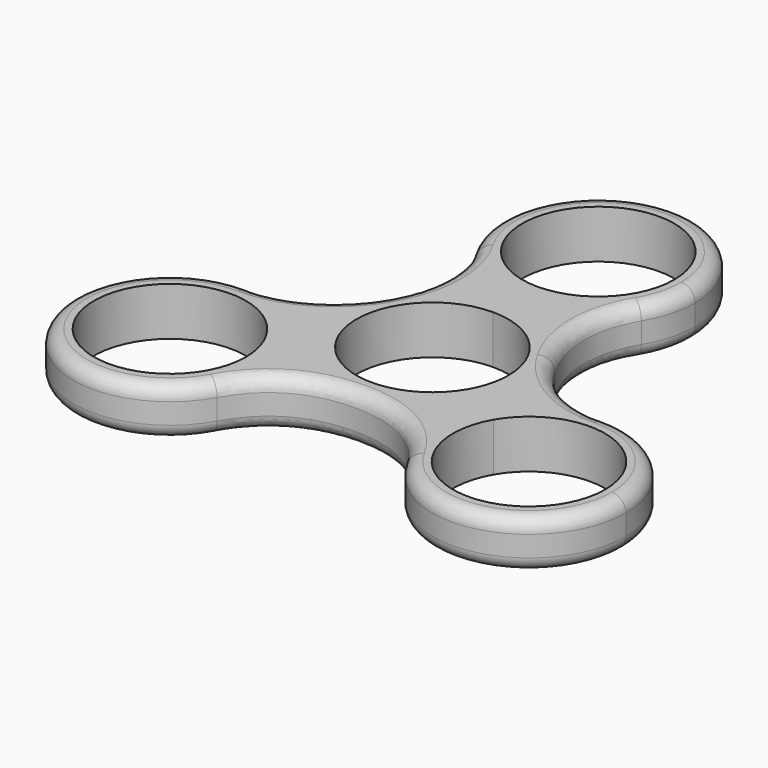
from build123d import *

# Parameters (mm, degrees)
F1_DEPTH = 7
F2_R     = 2


with BuildPart() as f1:
    # F0 (on Top) → F1 (new body)
    with BuildSketch(Plane.XY):
        with BuildLine():
            ThreePointArc((-11.9807621135, -15), (-12.4578005455, -11.3765333686), (-13.8564064606, -8))
            ThreePointArc((-13.8564064606, -8), (-18.8749387967, -2.9373603639), (-25.7357641151, -1.0021438791))
            ThreePointArc((-25.7357641151, -1.0021438791), (-38.1051177665, -22), (-13.7357641151, -21.7867535699))
            ThreePointArc((-13.7357641151, -21.7867535699), (-12.4266119746, -18.5049984324), (-11.9807621135, -15))
        make_face()
        with BuildLine():
            ThreePointArc((-14.9807621135, -15), (-36.6059462027, -17.8470094961), (-16.4544826719, -9.5))
            ThreePointArc((-16.4544826719, -9.5), (-15.3555780244, -12.1529905039), (-14.9807621135, -15))
        make_face(mode=Mode.SUBTRACT)
        with BuildLine():
            ThreePointArc((-9.5262794416, -5.5), (-9.5262794416, 5.5), (0, 11))
            Line((0, 11), (0, 14))
            ThreePointArc((0, 14), (-7.0000000057, 12.1243556497), (-12.1243556595, 6.9999999886))
            ThreePointArc((-12.1243556595, 6.9999999886), (-14, -6.6e-09), (-12.124355653, -7))
            Line((-12.124355653, -7), (-9.5262794416, -5.5))
        make_face()
        with BuildLine():
            Line((-13.8564064606, -8), (-12.124355653, -7))
            ThreePointArc((-12.124355653, -7), (-14, -6.6e-09), (-12.1243556595, 6.9999999886))
            add(Edge.make_bspline(
                [(-12.124355653, 7), (-14.8604643909, 2.2609206509), (-19.9785749652, -1.1029092968), (-25.7357641151, -1.0021438791)],
                knots=[0.5, 0.5, 0.5, 0.5, 1, 1, 1, 1], degree=3))
            ThreePointArc((-25.7357641151, -1.0021438791), (-18.8749387967, -2.9373603639), (-13.8564064606, -8))
        make_face()
        with BuildLine():
            Line((12.124355653, -7), (9.5262794416, -5.5))
            ThreePointArc((9.5262794416, -5.5), (0, -11), (-9.5262794416, -5.5))
            Line((-9.5262794416, -5.5), (-12.124355653, -7))
            ThreePointArc((-12.124355653, -7), (-6.9999999959, -12.1243556553), (9.4e-09, -14))
            ThreePointArc((9.4e-09, -14), (7.0000000041, -12.1243556506), (12.124355653, -7))
        make_face()
        with BuildLine():
            ThreePointArc((9.4e-09, -14), (-6.9999999959, -12.1243556553), (-12.124355653, -7))
            Line((-12.124355653, -7), (-13.8564064606, -8))
            ThreePointArc((-13.8564064606, -8), (-12.4578005455, -11.3765333686), (-11.9807621135, -15))
            ThreePointArc((-11.9807621135, -15), (-12.4266119746, -18.5049984324), (-13.7357641151, -21.7867535699))
            add(Edge.make_bspline(
                [(-13.7357641151, -21.7867535699), (-10.4992239257, -15.947226949), (-5.2496119628, -14), (0, -14)],
                knots=[0, 0, 0, 0, 0.5, 0.5, 0.5, 0.5], degree=3))
        make_face()
        with BuildLine():
            Line((13.8564064606, -8), (12.124355653, -7))
            ThreePointArc((12.124355653, -7), (7.0000000041, -12.1243556506), (9.4e-09, -14))
            add(Edge.make_bspline(
                [(0, -14), (5.2496119628, -14), (10.4992239257, -15.947226949), (13.7357641151, -21.7867535699)],
                knots=[0.5, 0.5, 0.5, 0.5, 1, 1, 1, 1], degree=3))
            ThreePointArc((13.7357641151, -21.7867535699), (11.9812980936, -14.8774963108), (13.8564064606, -8))
        make_face()
        with BuildLine():
            ThreePointArc((0, 11), (7.7781745931, 7.7781745931), (11, 0))
            ThreePointArc((11, 0), (10.6251840892, -2.8470094961), (9.5262794416, -5.5))
            Line((9.5262794416, -5.5), (12.124355653, -7))
            ThreePointArc((12.124355653, -7), (13.522961568, -3.6234666314), (14, 0))
            ThreePointArc((14, 0), (13.5229615737, 3.6234666105), (12.1243556746, 6.9999999625))
            ThreePointArc((12.1243556746, 6.9999999625), (7.0000000188, 12.1243556422), (0, 14))
            Line((0, 14), (0, 11))
        make_face()
        with BuildLine():
            ThreePointArc((25.7357641151, -1.0021438791), (18.8749387967, -2.9373603639), (13.8564064606, -8))
            ThreePointArc((13.8564064606, -8), (11.9812980936, -14.8774963108), (13.7357641151, -21.7867535699))
            ThreePointArc((13.7357641151, -21.7867535699), (29.4857605459, -28.5541501389), (39.9807621135, -15))
            ThreePointArc((39.9807621135, -15), (35.7932548657, -5.0142608692), (25.7357641151, -1.0021438791))
        make_face()
        with BuildLine():
            ThreePointArc((36.9807621135, -15), (23.1337526174, -25.6251840892), (16.4544826719, -9.5))
            ThreePointArc((16.4544826719, -9.5), (28.8277716097, -4.3748159108), (36.9807621135, -15))
        make_face(mode=Mode.SUBTRACT)
        with BuildLine():
            ThreePointArc((14, 0), (13.522961568, -3.6234666314), (12.124355653, -7))
            Line((12.124355653, -7), (13.8564064606, -8))
            ThreePointArc((13.8564064606, -8), (18.8749387967, -2.9373603639), (25.7357641151, -1.0021438791))
            add(Edge.make_bspline(
                [(12.124355653, 7), (14.8196855562, 2.3315516644), (19.6421453279, -1.108797669), (25.7357641151, -1.0021438791)],
                knots=[0.5, 0.5, 0.5, 0.5, 1, 1, 1, 1], degree=3))
            ThreePointArc((12.1243556746, 6.9999999625), (13.5229615737, 3.6234666105), (14, 0))
        make_face()
        with BuildLine():
            Line((0, 16), (0, 14))
            ThreePointArc((0, 14), (7.0000000188, 12.1243556422), (12.1243556746, 6.9999999625))
            add(Edge.make_bspline(
                [(12, 22.7888974491), (8.8608257149, 17.5649956733), (9.4290257497, 11.6684483356), (12.124355653, 7)],
                knots=[0, 0, 0, 0, 0.5, 0.5, 0.5, 0.5], degree=3))
            ThreePointArc((12, 22.7888974491), (6.8936407031, 17.8148566748), (0, 16))
        make_face()
        with BuildLine():
            ThreePointArc((-12.1243556595, 6.9999999886), (-7.0000000057, 12.1243556497), (0, 14))
            Line((0, 14), (0, 16))
            ThreePointArc((0, 16), (-6.8936407031, 17.8148566748), (-12, 22.7888974491))
            add(Edge.make_bspline(
                [(-12, 22.7888974491), (-9.0341400135, 17.8534080997), (-9.3882469151, 11.7390793491), (-12.124355653, 7)],
                knots=[0, 0, 0, 0, 0.5, 0.5, 0.5, 0.5], degree=3))
        make_face()
        with BuildLine():
            ThreePointArc((-12, 22.7888974491), (-6.8936407031, 17.8148566748), (0, 16))
            ThreePointArc((0, 16), (6.8936407031, 17.8148566748), (12, 22.7888974491))
            ThreePointArc((12, 22.7888974491), (13.4907375632, 26.2583426132), (14, 30))
            ThreePointArc((14, 30), (-3.7416573868, 43.4907375632), (-12, 22.7888974491))
        make_face()
        with BuildLine():
            ThreePointArc((11, 30), (7.7781745931, 22.2218254069), (0, 19))
            ThreePointArc((0, 19), (-7.7781745931, 37.7781745931), (11, 30))
        make_face(mode=Mode.SUBTRACT)
    extrude(amount=F1_DEPTH)

    # F2
    f2_edges = [f1.edges().sort_by_distance(p)[0] for p in [
        (-38.105118, -22, 0),
        (-38.105118, -22, 7),
    ]]
    fillet(f2_edges, radius=F2_R)


solid = f1.part
